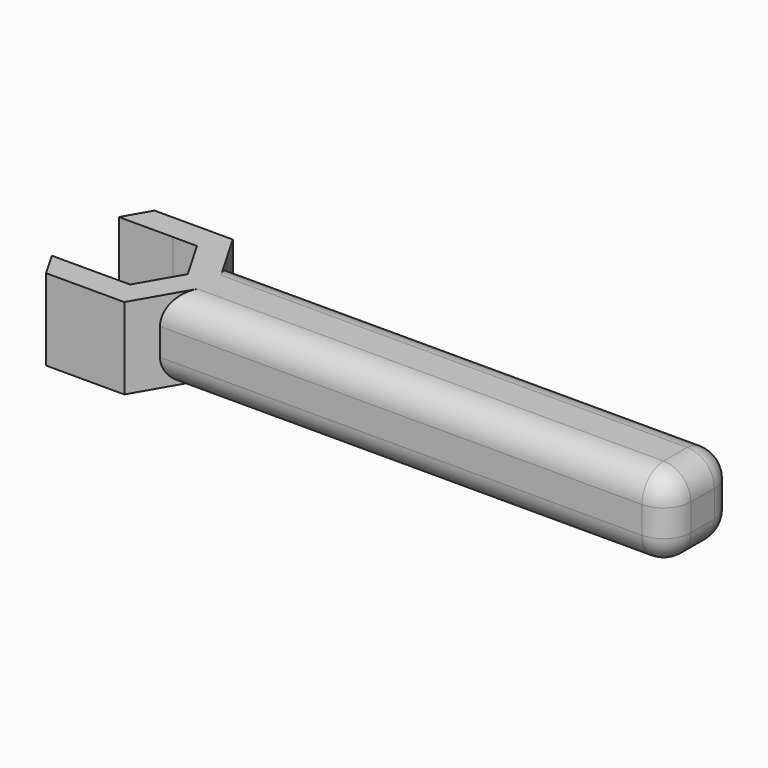
from build123d import *

# Parameters (mm, degrees)
F1_DEPTH     = 15.24
F2_R         = 5.08
F3_R         = 5.08
F4_R         = 5.08
F5_S3_W      = 5.08
F5_S3_H      = 5.08
F5_T4_DEPTH  = 5.08
F5_T10_DEPTH = 102.9839018281


# Not quite as in the source:
# - a fillet or chamfer that OpenCascade refuses, or shapes differently, is made with other operations: its cross-section is extruded or revolved along the edge and cut away or added


with BuildPart() as f1:
    # F0 (on Top) → F1 (new body)
    with BuildSketch(Plane.XY):
        Polygon((-45.1973650922, 20.5321404808), (-35.0638359103, 20.5321404808), (-24.9303067284, 20.5321404808), (-27.7331978752, 25.3868903553), (-42.3944739453, 25.3868903553), align=None)
        Polygon((-24.9303067284, 20.5321404808), (-35.0638359103, 20.5321404808), (-35.0638359103, 20.5181515061), (-30.5441655604, 20.5181515061), (-26.0244952105, 12.6898528267), (-30.5441655604, 4.8615541473), (-35.0638359103, 4.8615541473), (-35.0638359103, 4.8475651727), (-24.9303067284, 4.8475651727), (-20.4025598402, 12.6898528267), align=None)
        Polygon((-27.7331978752, -0.0071847018), (-24.9303067284, 4.8475651727), (-35.0638359103, 4.8475651727), (-45.1973650922, 4.8475651727), (-42.3944739453, -0.0071847018), align=None)
        Polygon((70.4335950998, 20.5321404808), (-24.9303067284, 20.5321404808), (-20.4025598402, 12.6898528267), (-24.9303067284, 4.8475651727), (70.4335950998, 4.8475651727), align=None)
    extrude(amount=F1_DEPTH)

    # F2
    f2_edges = [f1.edges().sort_by_distance(p)[0] for p in [
        (70.433595, 20.53214, 7.62),
        (70.433595, 12.689853, 15.24),
    ]]
    fillet(f2_edges, radius=F2_R)

    # F3
    f3_edges = [f1.edges().sort_by_distance(p)[0] for p in [
        (70.433595, 10.149853, 0),
    ]]
    fillet(f3_edges, radius=F3_R)

    # F4
    f4_edges = [f1.edges().sort_by_distance(p)[0] for p in [
        (70.433595, 4.847565, 7.62),
    ]]
    fillet(f4_edges, radius=F4_R)

    # F5: fillet of radius 5.08 on 1 edges, made by hand


with BuildPart() as f5_tool2:
    # F5_s3 → F5_t4 (new body)
    with BuildSketch(Plane.XY.offset(10.16)):
        with Locations((67.8935950998, 17.9921404808)):
            Rectangle(F5_S3_W, F5_S3_H)
    extrude(amount=F5_T4_DEPTH)

    # F5_s5 → F5_t6 (revolve, cut)
    with BuildSketch(Plane(origin=(65.3535950998, 15.4521404808, 10.16), x_dir=(-0.7071067812, -0.7071067812, 0), z_dir=(-0.7071067812, 0.7071067812, 0))):
        with BuildLine():
            ThreePointArc((0, -5.08), (5.08, 0), (0, 5.08))
            Line((0, 5.08), (0, -5.08))
        make_face()
    revolve(axis=Axis((65.3535950998, 15.4521404808, 10.16), (0, 0, 1)), mode=Mode.SUBTRACT)


with BuildPart() as f1_1:
    add(f1.part)

    # F5_t1: cut F5_tool2
    add(f5_tool2.part, mode=Mode.SUBTRACT)


with BuildPart() as f5_tool8:
    # F5_s9 → F5_t10 (new body)
    with BuildSketch(Plane.YZ.offset(65.3535950998)):
        with BuildLine():
            ThreePointArc((15.4521404808, 15.24), (19.0442429292, 13.7521024484), (20.5321404808, 10.16))
            Line((20.5321404808, 10.16), (20.5321404808, 15.24))
            Line((20.5321404808, 15.24), (15.4521404808, 15.24))
        make_face()
    extrude(amount=-F5_T10_DEPTH)

    split(bisect_by=Plane(origin=(-9.8070524211, -5.6621043553, 0), x_dir=(0, 0, 1), z_dir=(0.8660254038, 0.5, 0)), keep=Keep.TOP)


with BuildPart() as f1_2:
    add(f1_1.part)

    # F5_t7: cut F5_tool8
    add(f5_tool8.part, mode=Mode.SUBTRACT)


solid = f1_2.part
